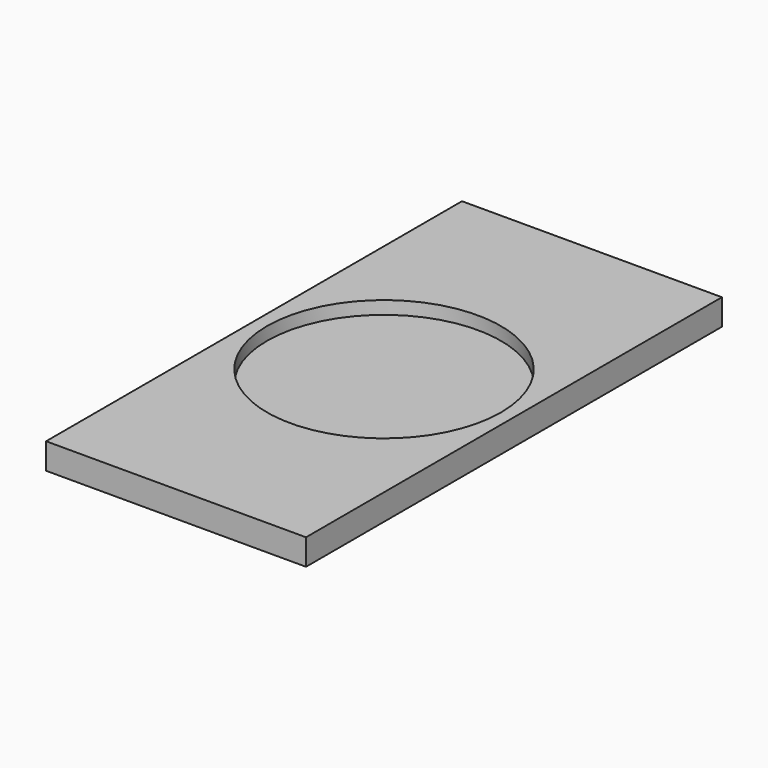
from build123d import *

# Parameters (mm, degrees)
F0_W     = 100
F0_H     = 200
F1_DEPTH = 10
F2_R     = 45
F3_DEPTH = 5


# Not quite as in the source:
# - a feature of the source that left no trace in its solid (it failed there, or was rolled back) is left out


with BuildPart() as f1:
    # F0 (on Top) → F1 (new body)
    with BuildSketch(Plane.XY):
        with Locations((1.6330834478, 54.0809953011)):
            Rectangle(F0_W, F0_H)
    extrude(amount=F1_DEPTH)

    # F2 (on face) → F3 (cut)
    with BuildSketch(Plane.XY.offset(10)):
        with Locations((1.6330834478, 54.0809953011)):
            Circle(F2_R)
    extrude(amount=-F3_DEPTH, mode=Mode.SUBTRACT)


solid = f1.part
